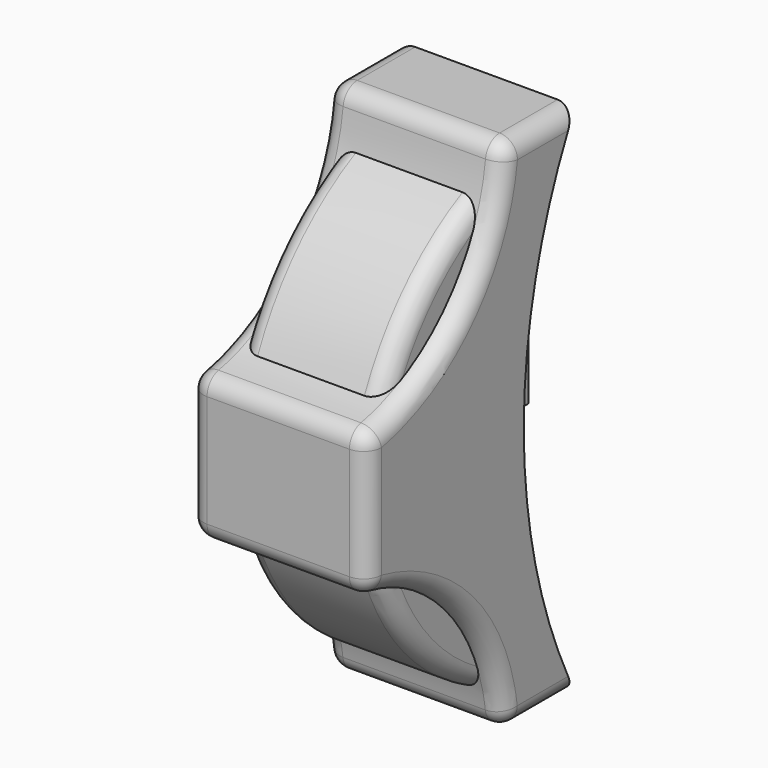
from build123d import *

# Parameters (mm, degrees)
F1_DEPTH = 5
F2_DEPTH = 4
F3_DEPTH = 1.25
F4_R     = 0.99999


# Not quite as in the source:
# - a fillet or chamfer is up to 0.001 mm smaller than in the source, because OpenCascade refuses the exact size


with BuildPart() as f1:
    # F0 (on Right) → F1 (new body, symmetric)
    with BuildSketch(Plane.YZ):
        with BuildLine():
            Line((-5, -14.5), (0, -14.5))
            ThreePointArc((0, -14.5), (-2.4437801933, -8.4394090773), (-3.5559108959, -2))
            ThreePointArc((-3.5559108959, -2), (-3.6208218956, 0), (-3.5559108959, 2))
            ThreePointArc((-3.5559108959, 2), (-2.4437801933, 8.4394090773), (0, 14.5))
            Line((0, 14.5), (-5, 14.5))
            ThreePointArc((-5, 14.5), (-5.1291387963, 13.134247874), (-5.4284954087, 11.7954643527))
            ThreePointArc((-5.4284954087, 11.7954643527), (-7.9929486595, 7.3268364788), (-12.3208218956, 4.5313814526))
            ThreePointArc((-12.3208218956, 4.5313814526), (-13.4564210039, 4.2033587599), (-14.6208218956, 4))
            Line((-14.6208218956, 4), (-14.6208218956, -4))
            ThreePointArc((-14.6208218956, -4), (-13.455545783, -4.2262388619), (-12.3208218956, -4.5747415742))
            ThreePointArc((-12.3208218956, -4.5747415742), (-7.768120381, -7.6921760362), (-5.2606798266, -12.6072783314))
            ThreePointArc((-5.2606798266, -12.6072783314), (-5.0898373373, -13.5480608471), (-5, -14.5))
        make_face()
    extrude(amount=F1_DEPTH, both=True)

    # F0 (on Right) → F2 (join, symmetric)
    with BuildSketch(Plane.YZ):
        with BuildLine():
            ThreePointArc((-12.3208218956, 4.5313814526), (-7.9929486595, 7.3268364788), (-5.4284954087, 11.7954643527))
            ThreePointArc((-5.4284954087, 11.7954643527), (-9.5138419457, 8.7698944978), (-12.3208218956, 4.5313814526))
        make_face()
        with BuildLine():
            ThreePointArc((-12.3208218956, -4.5747415742), (-9.56666639, -9.2729954865), (-5.2606798266, -12.6072783314))
            ThreePointArc((-5.2606798266, -12.6072783314), (-7.768120381, -7.6921760362), (-12.3208218956, -4.5747415742))
        make_face()
    extrude(amount=F2_DEPTH, both=True)

    # F0 (on Right) → F3 (join, symmetric)
    with BuildSketch(Plane.YZ):
        with BuildLine():
            ThreePointArc((-3.5559108959, 2), (-3.6208218956, 0), (-3.5559108959, -2))
            Line((-3.5559108959, -2), (1.3791781044, -2))
            Line((1.3791781044, -2), (1.3791781044, 2))
            Line((1.3791781044, 2), (-3.5559108959, 2))
        make_face()
    extrude(amount=F3_DEPTH, both=True)

    # F4 (radius 1 in the source; OpenCascade refuses exactly that, so slightly less here)
    f4_edges = [f1.edges().sort_by_distance(p)[0] for p in [
        (5, -14.620822, 0),
        (5, -7.992949, 7.326836),
        (5, -7.76812, -7.692176),
        (-5, -7.992949, 7.326836),
        (-5, -14.620822, 0),
        (-5, -7.76812, -7.692176),
        (-2.5, -5, 14.5),
        (2.5, -5, 14.5),
        (-2.5, -5, -14.5),
        (2.5, -5, -14.5),
        (-5, -2.5, 14.5),
        (5, -2.5, 14.5),
        (-5, -2.5, -14.5),
        (5, -2.5, -14.5),
        (4, -9.566666, -9.272995),
        (-4, -9.566666, -9.272995),
        (4, -9.513842, 8.769894),
        (-4, -9.513842, 8.769894),
        (-2.5, -14.620822, 4),
        (2.5, -14.620822, 4),
        (-2.5, -14.620822, -4),
        (2.5, -14.620822, -4),
    ]]
    fillet(f4_edges, radius=F4_R)


solid = f1.part
